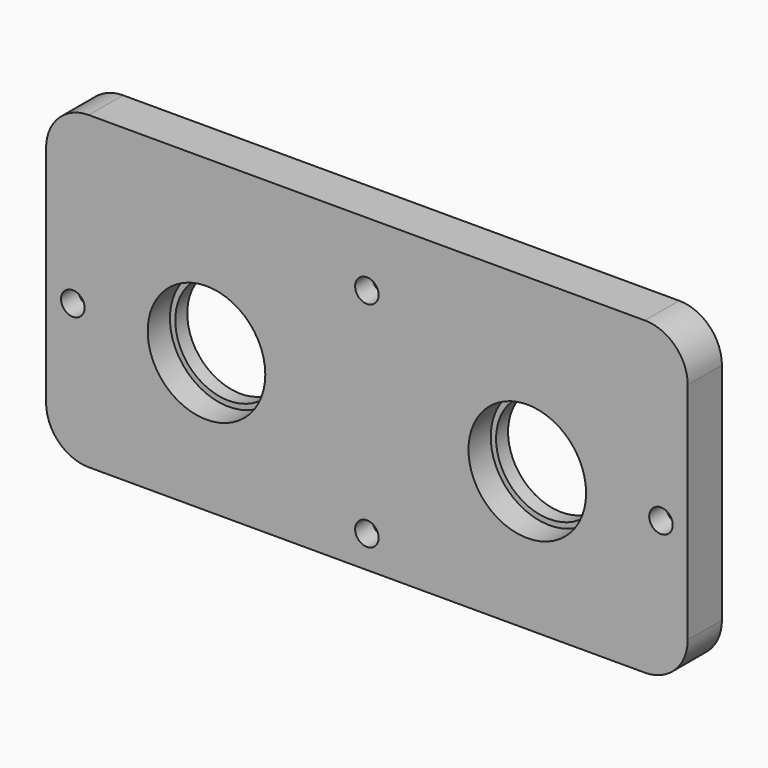
from build123d import *

# Parameters (mm, degrees)
F0_W      = 300
F0_H      = 160
F1_DEPTH  = 10
F2_R      = 25
F3_DEPTH  = 20.001
F4_R      = 5.5
F5_DEPTH  = 10
F6_W      = 300
F6_H      = 15
F7_DEPTH  = 20.001
F8_R      = 20
F9_R      = 27.5
F10_DEPTH = 13


with BuildPart() as f1:
    # F0 (on Front) → F1 (new body, symmetric)
    with BuildSketch(Plane.XZ):
        Rectangle(F0_W, F0_H)
    extrude(amount=F1_DEPTH, both=True)

    # F2 (on face) → F3 (cut, through all)
    with BuildSketch(Plane.XZ.offset(10)):
        with Locations((-75, 0)):
            Circle(F2_R)
        with Locations((75, 0)):
            Circle(F2_R)
    extrude(amount=-F3_DEPTH, mode=Mode.SUBTRACT)

    # F4 (on face) → F5 (cut)
    with BuildSketch(Plane.XZ.offset(10)):
        with Locations((-137.5, 0)):
            Circle(F4_R)
        with Locations((0, 50)):
            Circle(F4_R)
        with Locations((137.5, 0)):
            Circle(F4_R)
        with Locations((0, -50)):
            Circle(F4_R)
    extrude(amount=-F5_DEPTH, mode=Mode.SUBTRACT)

    # F6 (on face) → F7 (cut, through all)
    with BuildSketch(Plane.XZ.offset(10)):
        with Locations((0, -72.5)):
            Rectangle(F6_W, F6_H)
    extrude(amount=-F7_DEPTH, mode=Mode.SUBTRACT)

    # F8
    f8_edges = [f1.edges().sort_by_distance(p)[0] for p in [
        (-150, 0, 80),
        (150, 0, 80),
        (-150, 0, -65),
        (150, 0, -65),
    ]]
    fillet(f8_edges, radius=F8_R)

    # F9 (on face) → F10 (cut)
    with BuildSketch(Plane.XZ.offset(10)):
        with Locations((-75, 0)):
            Circle(F9_R)
        with Locations((75, 0)):
            Circle(F9_R)
    extrude(amount=-F10_DEPTH, mode=Mode.SUBTRACT)


solid = f1.part
